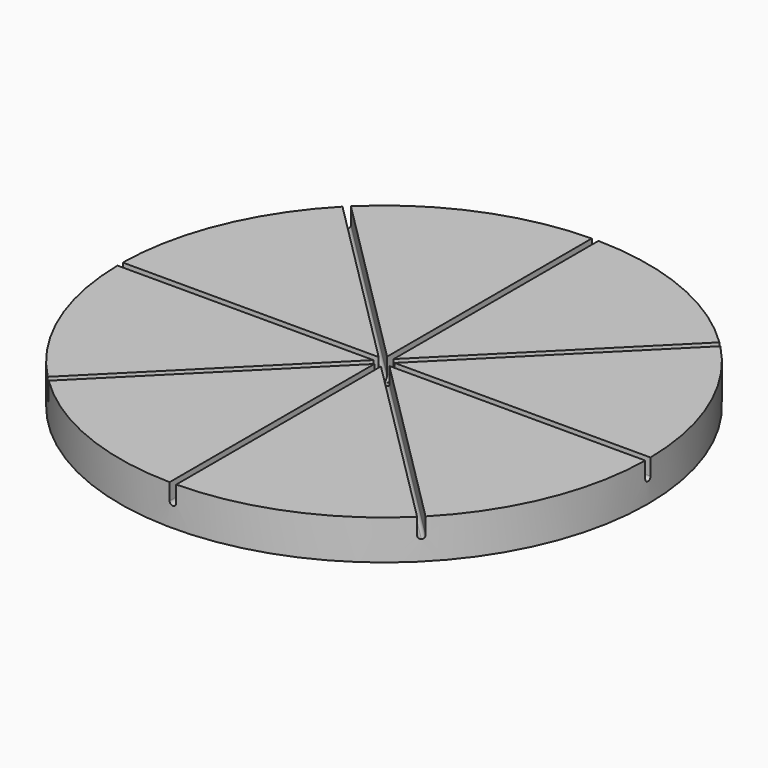
from build123d import *

# Parameters (mm, degrees)
F0_R     = 254
F1_DEPTH = 38.1
F3_DEPTH = 19.05
F4_DEPTH = 19.05
F5_R     = 3.175
F5_R_2   = 3.17499


# Not quite as in the source:
# - a fillet or chamfer is up to 0.001 mm smaller than in the source, because OpenCascade refuses the exact size


with BuildPart() as f1:
    # F0 (on Top) → F1 (new body)
    with BuildSketch(Plane.XY):
        Circle(F0_R)
    extrude(amount=F1_DEPTH)

    # F2 (on face) → F3 (cut)
    with BuildSketch(Plane.XY.offset(38.1)):
        Polygon((-3.175, -7.6651280605), (-3.175, -254), (3.175, -254), (3.175, -7.6651280605), (0, -4.4901280605), align=None)
        Polygon((-177.3600583911, -181.8501864516), (-3.175, -7.6651280605), (-3.175, -3.175), (-7.6651280605, -3.175), (-181.8501864517, -177.3600583911), align=None)
        Polygon((-3.175, -3.175), (-3.175, -7.6651280605), (0, -4.4901280605), (-1.3151280605, -3.175), align=None)
        Polygon((0, -4.4901280605), (3.175, -7.6651280605), (3.175, -3.175), (1.3151280605, -3.175), align=None)
        Polygon((3.175, -3.175), (3.175, -7.6651280605), (177.3600583911, -181.8501864517), (181.8501864517, -177.3600583911), (7.6651280605, -3.175), align=None)
        Polygon((-7.6651280605, -3.175), (-3.175, -3.175), (-3.175, -1.3151280605), (-4.4901280605, 0), align=None)
        Polygon((3.175, -1.3151280605), (3.175, -3.175), (7.6651280605, -3.175), (4.4901280605, 0), align=None)
        Polygon((-254, -3.175), (-7.6651280605, -3.175), (-4.4901280605, 0), (-7.6651280605, 3.175), (-254, 3.175), align=None)
        Polygon((4.4901280605, 0), (7.6651280605, -3.175), (254, -3.175), (254, 3.175), (7.6651280605, 3.175), align=None)
        Polygon((-4.4901280605, 0), (-3.175, 1.3151280605), (-3.175, 3.175), (-7.6651280605, 3.175), align=None)
        Polygon((3.175, 3.175), (3.175, 1.3151280605), (4.4901280605, 0), (7.6651280605, 3.175), align=None)
        Polygon((-7.6651280605, 3.175), (-3.175, 3.175), (-3.175, 7.6651280605), (-177.3600583911, 181.8501864517), (-181.8501864517, 177.3600583911), align=None)
        Polygon((-3.175, 7.6651280605), (-3.175, 3.175), (-1.3151280605, 3.175), (0, 4.4901280605), align=None)
        Polygon((1.3151280605, 3.175), (3.175, 3.175), (3.175, 7.6651280605), (0, 4.4901280605), align=None)
        Polygon((3.175, 7.6651280605), (3.175, 3.175), (7.6651280605, 3.175), (181.8501864517, 177.3600583911), (177.3600583911, 181.8501864517), align=None)
        Polygon((-3.175, 254), (-3.175, 7.6651280605), (0, 4.4901280605), (3.175, 7.6651280605), (3.175, 254), align=None)
    extrude(amount=-F3_DEPTH, mode=Mode.SUBTRACT)

    # F4 (cut, through all): a face of the model
    f4_faces = [f1.faces().sort_by_distance(p)[0] for p in [
        (0, 0, 38.1),
    ]]
    extrude(f4_faces, amount=-F4_DEPTH, mode=Mode.SUBTRACT)

    # F5 (call 1 of 8: OpenCascade refuses the feature's edges together)
    f5_edges = [f1.edges().sort_by_distance(p)[0] for p in [
        (3.175, 130.822642, 19.05),
        (90.260513, 94.750641, 19.05),
    ]]
    fillet(f5_edges, radius=F5_R)

    # F5#2 (call 2 of 8) (radius 3.175 in the source; OpenCascade refuses exactly that, so slightly less here)
    f5_2_edges = [f1.edges().sort_by_distance(p)[0] for p in [
        (-3.175, 130.822642, 19.05),
        (-90.260513, 94.750641, 19.05),
    ]]
    fillet(f5_2_edges, radius=F5_R_2)

    # F5#3 (call 3 of 8)
    f5_3_edges = [f1.edges().sort_by_distance(p)[0] for p in [
        (-130.822642, 3.175, 19.05),
        (-94.750641, 90.260513, 19.05),
    ]]
    fillet(f5_3_edges, radius=F5_R)

    # F5#4 (call 4 of 8)
    f5_4_edges = [f1.edges().sort_by_distance(p)[0] for p in [
        (-3.175, -130.822642, 19.05),
        (-90.260513, -94.750641, 19.05),
    ]]
    fillet(f5_4_edges, radius=F5_R)

    # F5#5 (call 5 of 8) (radius 3.175 in the source; OpenCascade refuses exactly that, so slightly less here)
    f5_5_edges = [f1.edges().sort_by_distance(p)[0] for p in [
        (-130.822642, -3.175, 19.05),
        (-94.750641, -90.260513, 19.05),
    ]]
    fillet(f5_5_edges, radius=F5_R_2)

    # F5#6 (call 6 of 8) (radius 3.175 in the source; OpenCascade refuses exactly that, so slightly less here)
    f5_6_edges = [f1.edges().sort_by_distance(p)[0] for p in [
        (3.175, -130.822642, 19.05),
        (90.260513, -94.750641, 19.05),
    ]]
    fillet(f5_6_edges, radius=F5_R_2)

    # F5#7 (call 7 of 8)
    f5_7_edges = [f1.edges().sort_by_distance(p)[0] for p in [
        (130.822642, -3.175, 19.05),
        (94.750641, -90.260513, 19.05),
    ]]
    fillet(f5_7_edges, radius=F5_R)

    # F5#8 (call 8 of 8) (radius 3.175 in the source; OpenCascade refuses exactly that, so slightly less here)
    f5_8_edges = [f1.edges().sort_by_distance(p)[0] for p in [
        (130.822642, 3.175, 19.05),
        (94.750641, 90.260513, 19.05),
    ]]
    fillet(f5_8_edges, radius=F5_R_2)


solid = f1.part
